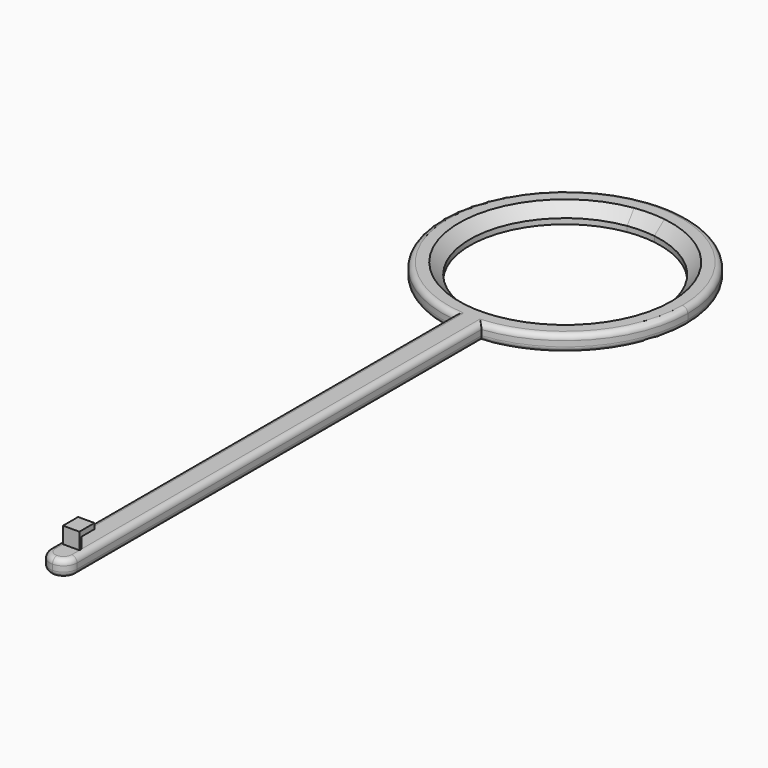
from build123d import *

# Parameters (mm, degrees)
F1_DEPTH = 3
F0_W     = 3
F0_H     = 0.2339549768
F2_DEPTH = 6
F3_W     = 3
F3_H     = 1
F4_DEPTH = 3
F5_R     = 0.99999
F6_SIZE  = 2


# Not quite as in the source:
# - a fillet or chamfer is up to 0.001 mm smaller than in the source, because OpenCascade refuses the exact size
# - a feature names something its author has since deleted; it is built from what else it names


with BuildPart() as f1:
    # F0 (on Top) → F1 (new body)
    with BuildSketch(Plane.XY):
        with BuildLine():
            Line((-2.5, 70), (2.5, 70))
            ThreePointArc((2.5, 70), (0, 70.139320225), (-2.5, 70))
        make_face()
        with BuildLine():
            ThreePointArc((22.5, 47.639320225), (16.7705098312, 62.639320225), (2.5, 70))
            Line((2.5, 70), (2.5, 64.9598283007))
            ThreePointArc((2.5, 64.9598283007), (13.2287565553, 59.0957594624), (17.5, 47.639320225))
            ThreePointArc((17.5, 47.639320225), (13.2287565553, 36.1828809876), (2.5, 30.3188121493))
            Line((2.5, 30.3188121493), (2.5, 25.27864045))
            ThreePointArc((2.5, 25.27864045), (16.7705098312, 32.639320225), (22.5, 47.639320225))
        make_face()
        with BuildLine():
            Line((-2.5, 64.9598283007), (-2.5, 70))
            ThreePointArc((-2.5, 70), (-22.5, 47.639320225), (-2.5, 25.27864045))
            Line((-2.5, 25.27864045), (-2.5, 30.3188121493))
            ThreePointArc((-2.5, 30.3188121493), (-17.5, 47.639320225), (-2.5, 64.9598283007))
        make_face()
        with BuildLine():
            Line((2.5, 64.9598283007), (2.5, 70))
            Line((2.5, 70), (-2.5, 70))
            Line((-2.5, 70), (-2.5, 64.9598283007))
            ThreePointArc((-2.5, 64.9598283007), (0, 65.139320225), (2.5, 64.9598283007))
        make_face()
        with BuildLine():
            Line((-2.5, 30.3188121493), (-2.5, 25.27864045))
            ThreePointArc((-2.5, 25.27864045), (0, 25.139320225), (2.5, 25.27864045))
            Line((2.5, 25.27864045), (2.5, 30.3188121493))
            ThreePointArc((2.5, 30.3188121493), (0, 30.139320225), (-2.5, 30.3188121493))
        make_face()
        with BuildLine():
            Line((-1.5, -65.5), (-2.5, -65.5))
            Line((-2.5, -65.5), (-2.5, -67.5))
            ThreePointArc((-2.5, -67.5), (-1.767766953, -69.267766953), (0, -70))
            ThreePointArc((0, -70), (1.767766953, -69.267766953), (2.5, -67.5))
            Line((2.5, -67.5), (2.5, -65.5))
            Line((2.5, -65.5), (1.5, -65.5))
            Line((1.5, -65.5), (1.5, -65.7339549768))
            Line((1.5, -65.7339549768), (-1.5, -65.7339549768))
            Line((-1.5, -65.7339549768), (-1.5, -65.5))
        make_face()
        with BuildLine():
            ThreePointArc((2.5, 25.27864045), (0, 25.139320225), (-2.5, 25.27864045))
            Line((-2.5, 25.27864045), (-2.5, -65.5))
            Line((-2.5, -65.5), (-1.5, -65.5))
            Line((-1.5, -65.5), (-1.5, -65.2660450232))
            Line((-1.5, -65.2660450232), (1.5, -65.2660450232))
            Line((1.5, -65.2660450232), (1.5, -65.5))
            Line((1.5, -65.5), (2.5, -65.5))
            Line((2.5, -65.5), (2.5, 25.27864045))
        make_face()
    extrude(amount=F1_DEPTH)

    # F0 (on Top) → F2 (join)
    with BuildSketch(Plane.XY):
        with Locations((0, -65.3830225116)):
            Rectangle(F0_W, F0_H)
        with Locations((0, -65.6169774884)):
            Rectangle(F0_W, F0_H)
    extrude(amount=F2_DEPTH)

    # F3 (on face) → F4 (join)
    with BuildSketch(Plane(origin=(0, -65.2660450232, 0), x_dir=(-1, 0, 0), z_dir=(0, 1, 0))):
        with Locations((0, 5.5)):
            Rectangle(F3_W, F3_H)
    extrude(amount=F4_DEPTH)

    # F5 (radius 1 in the source; OpenCascade refuses exactly that, so slightly less here)
    f5_edges = [f1.edges().sort_by_distance(p)[0] for p in [
        (0, 70.13932, 3),
        (0, 70.13932, 0),
        (2.5, -21.11068, 0),
        (2.5, -21.11068, 3),
        (-2.5, -21.11068, 3),
        (-2.5, -21.11068, 0),
    ]]
    fillet(f5_edges, radius=F5_R)

    # F6
    f6_edges = [f1.edges().sort_by_distance(p)[0] for p in [
        (-2.5, 64.959828, 3),
    ]]
    chamfer(f6_edges, length=F6_SIZE)


solid = f1.part
